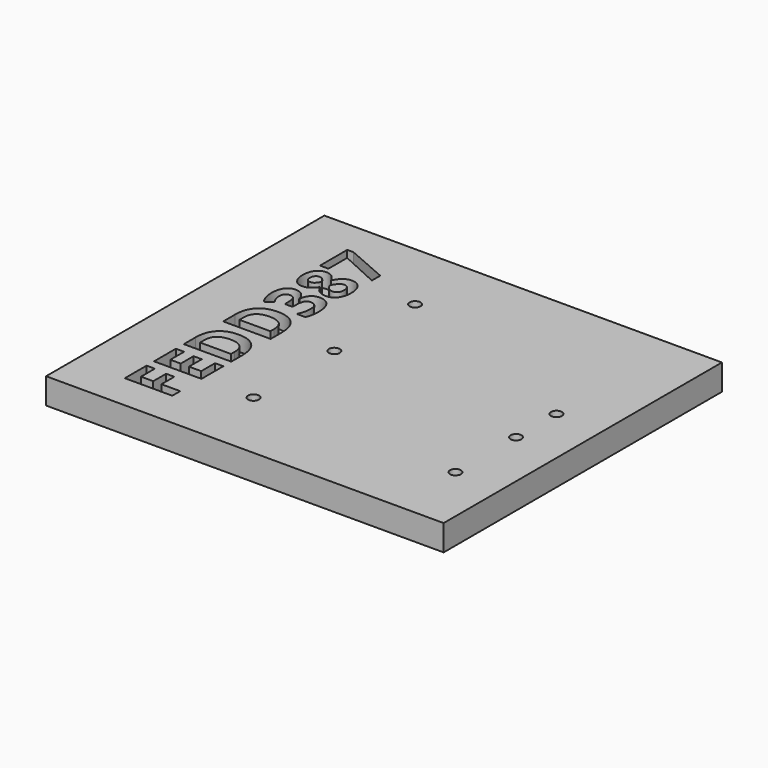
from build123d import *

# Parameters (mm, degrees)
F0_W         = 40
F0_H         = 35
F1_DEPTH     = 2.6
F2_TEXT_SIZE = 6.6897347174
F3_DEPTH     = 1.5
F4_R         = 0.55
F4_R_2       = 0.5500012936
F5_DEPTH     = 2.6


# Not quite as in the source:
# - Text() gives the source's letters only with a copy of the font that has no kerning and outlines rounded to 1/6400 em; it was checked with that copy


with BuildPart() as f1:
    # F0 (on Top) → F1 (new body)
    with BuildSketch(Plane.XY):
        with Locations((-23.1587231159, -4.1649090929)):
            Rectangle(F0_W, F0_H)
    extrude(amount=F1_DEPTH)

    # F2 (on face) → F3 (cut)
    with BuildSketch(Plane.XY.offset(2.6)):
        with Locations(Location((-33.3421141194, -18.6649090929), (0, 0, 90))):
            Text('FEDD387', F2_TEXT_SIZE, font='Open Sans', font_style=FontStyle.BOLD, text_align=(TextAlign.LEFT, TextAlign.BOTTOM))
    extrude(amount=-F3_DEPTH, mode=Mode.SUBTRACT)

    # F4 (on face) → F5 (cut, through all)
    with BuildSketch(Plane.XY.offset(2.6)):
        with Locations((-28.1587231159, 5.9950909071)):
            Circle(F4_R)
        with Locations((-28.1587231159, -4.1649090929)):
            Circle(F4_R)
        with Locations((-28.1587231159, -14.3249090929)):
            Circle(F4_R)
        with Locations((-7.8387231159, -1.6249090929)):
            Circle(F4_R)
        with Locations((-7.8387231159, -6.7049090929)):
            Circle(F4_R_2)
        with Locations((-7.8387231159, -14.3249090929)):
            Circle(F4_R)
    extrude(amount=-F5_DEPTH, mode=Mode.SUBTRACT)


solid = f1.part
